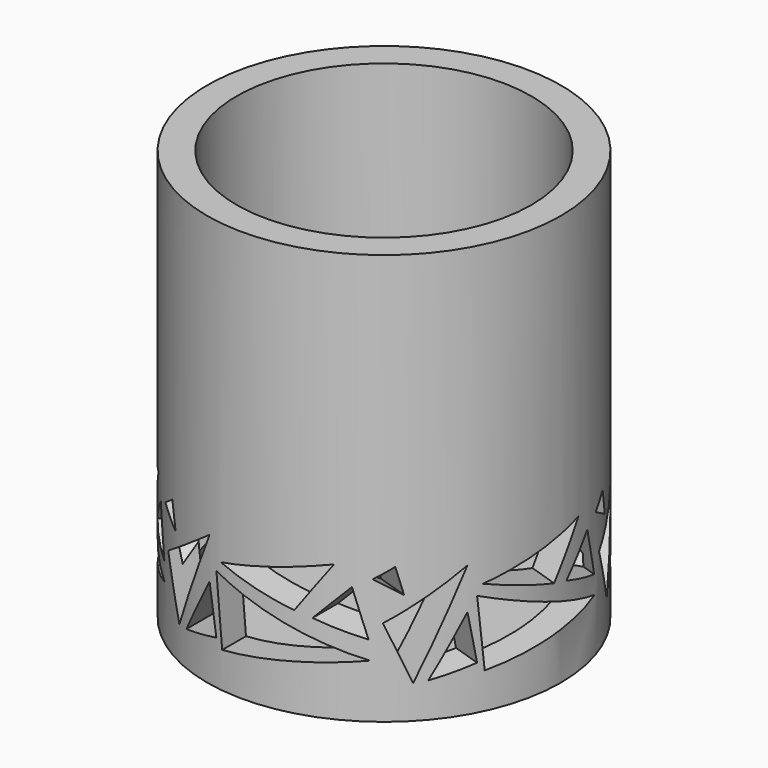
from build123d import *

# Parameters (mm, degrees)
F3_DEPTH        = 30.001
F3_COPIES_COUNT = 5


# Not quite as in the source:
# - a pattern or mirror of a feature is missing from the dataset's text; its kind, count and spacing are read off the source's solid


with BuildPart() as f1:
    # F0 (on Front) → F1 (revolve)
    with BuildSketch(Plane.XZ):
        Polygon((0, 5), (0, 0), (30, 0), (30, 69.708), (25, 69.708), (25, 5), align=None)
    revolve(axis=Axis((0, 0, 2.5), (0, 0, 1)))

    # F2 (on Front) → F3 (cut, through all)
    with BuildSketch(Plane.XZ):
        Polygon((-13.1414057687, 5.6357062422), (-6.0895560309, 22.2882665694), (-16.6248492897, 14.7266443819), align=None)
        Polygon((17.2750037163, 9.1191502288), (-4.7301636077, 17.4454301596), (-3.6256567109, 6.0605164617), align=None)
        Polygon((17.1050801873, 12.2627457604), (15.2359157801, 19.9942905456), (10.3930793703, 14.7266443819), align=None)
        Polygon((7.9291807488, 15.406341292), (13.1118651479, 23.1378860772), (-3.8805431686, 19.059708342), align=None)
        Polygon((-15.2222189495, 23.1378860772), (-17.729356885, 21.2687216699), (-14.2069354317, 18.9075378159), align=None)
        Polygon((-4.7301636077, 7.4606905805), (-6.0895560309, 15.3213795274), (-11.2722394988, 5.890592467), align=None)
    f3 = extrude(amount=F3_DEPTH, mode=Mode.SUBTRACT)

    # F3_copies: F3 ×5 about axis
    f3_copies_axis = Axis((0, 0, 0), (0, 0, 1))
    for i in range(1, F3_COPIES_COUNT):
        add(f3.rotate(f3_copies_axis, i * 360 / F3_COPIES_COUNT), mode=Mode.SUBTRACT)


solid = f1.part
